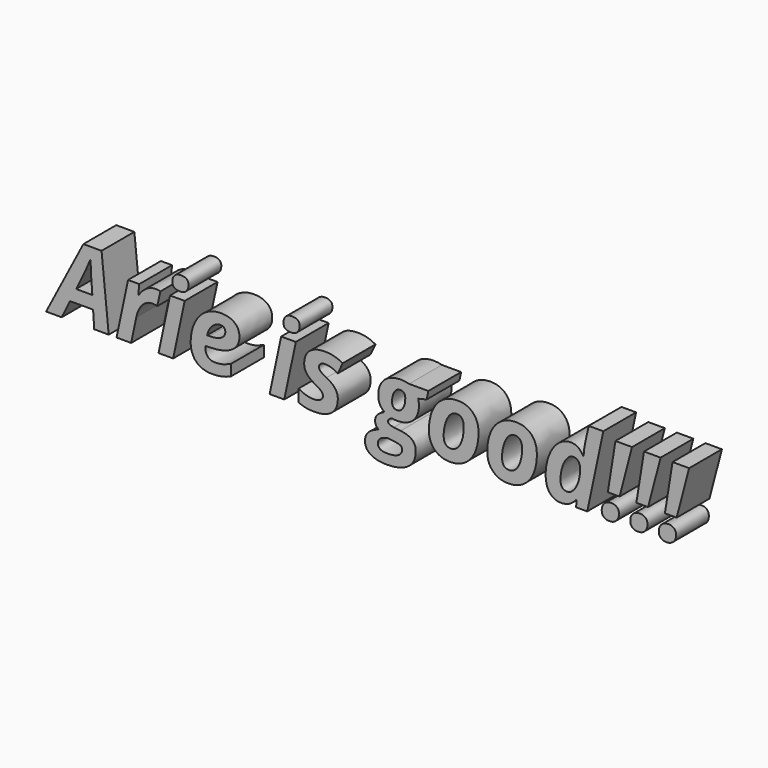
from build123d import *

# Parameters (mm, degrees)
F0_TEXT_SIZE = 60.8063820336
F1_DEPTH     = 25


# Not quite as in the source:
# - Text() gives the source's letters only with a copy of the font that has no kerning and outlines rounded to 1/6400 em; it was checked with that copy


with BuildPart() as f1:
    # F0 (on Front) → F1 (new body)
    with BuildSketch(Plane.XZ):
        with Locations((-34.9694080651, -18.723776564)):
            Text('Arie is good!!!', F0_TEXT_SIZE, font='Open Sans', font_style=FontStyle.BOLDITALIC, text_align=(TextAlign.LEFT, TextAlign.BOTTOM))
    extrude(amount=F1_DEPTH)


solid = f1.part
